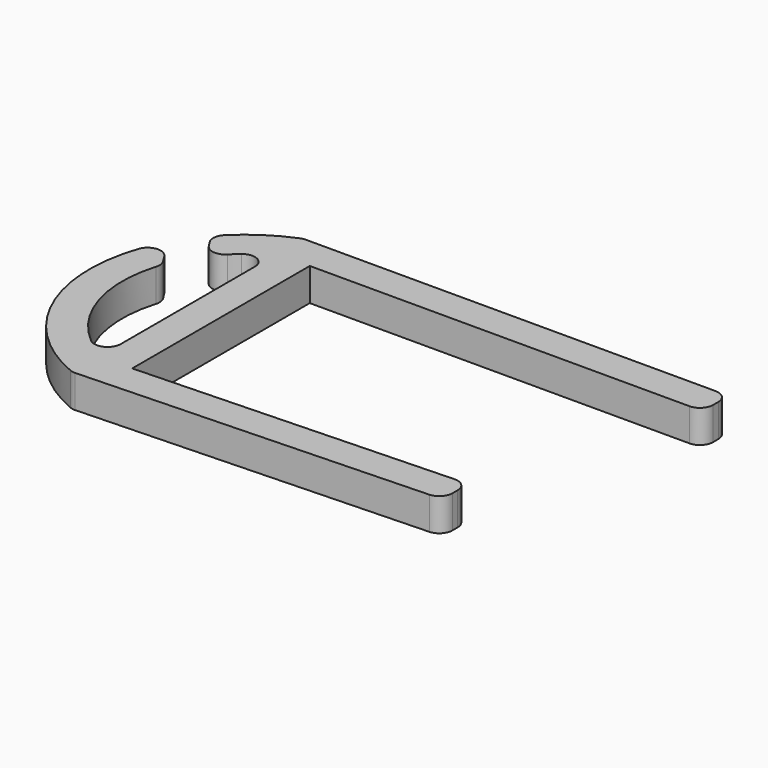
from build123d import *

# Parameters (mm, degrees)
F1_DEPTH = 5
F2_R     = 2


with BuildPart() as f1:
    # F0 (on Top) → F1 (new body)
    with BuildSketch(Plane.XY):
        Polygon((49.969541351, 1.7449748351), (0, 0), (0, 33.9), (60, 33.9), (60, 38.9), (-5, 38.9), (-5, 33.4082755117), (-5, 0.3140729194), (-5, -5.177651569), (49.969541351, -3.2580728864), align=None)
        with BuildLine():
            Line((-5, 33.4082755117), (-5, 38.9))
            ThreePointArc((-5, 38.9), (-9.8858414628, 36.2755829056), (-14.0276237399, 32.5871345254))
            Line((-14.0276237399, 32.5871345254), (-11.1949861447, 28.1640846398))
            ThreePointArc((-11.1949861447, 28.1640846398), (-8.385603023, 31.1265256497), (-5, 33.4082755117))
        make_face()
        with BuildLine():
            ThreePointArc((-17.1309979161, 28.161794916), (-18.5720640821, 8.7607088143), (-5, -5.177651569))
            Line((-5, -5.177651569), (-5, 0.3140729194))
            ThreePointArc((-5, 0.3140729194), (-13.7193681247, 10.061847649), (-13.9141851806, 23.1388709719))
            Line((-13.9141851806, 23.1388709719), (-17.1309979161, 28.161794916))
        make_face()
    extrude(amount=F1_DEPTH)

    # F2
    f2_edges = [f1.edges().sort_by_distance(p)[0] for p in [
        (49.969541, 1.744975, 2.5),
        (49.969541, -3.258073, 2.5),
        (-5, -5.177652, 2.5),
        (-5, 0.314073, 2.5),
        (-5, 33.408276, 2.5),
        (60, 33.9, 2.5),
        (-17.130998, 28.161795, 2.5),
        (-14.027624, 32.587135, 2.5),
        (-13.914185, 23.138871, 2.5),
        (-11.194986, 28.164085, 2.5),
        (-5, 38.9, 2.5),
        (60, 38.9, 2.5),
    ]]
    fillet(f2_edges, radius=F2_R)


solid = f1.part
